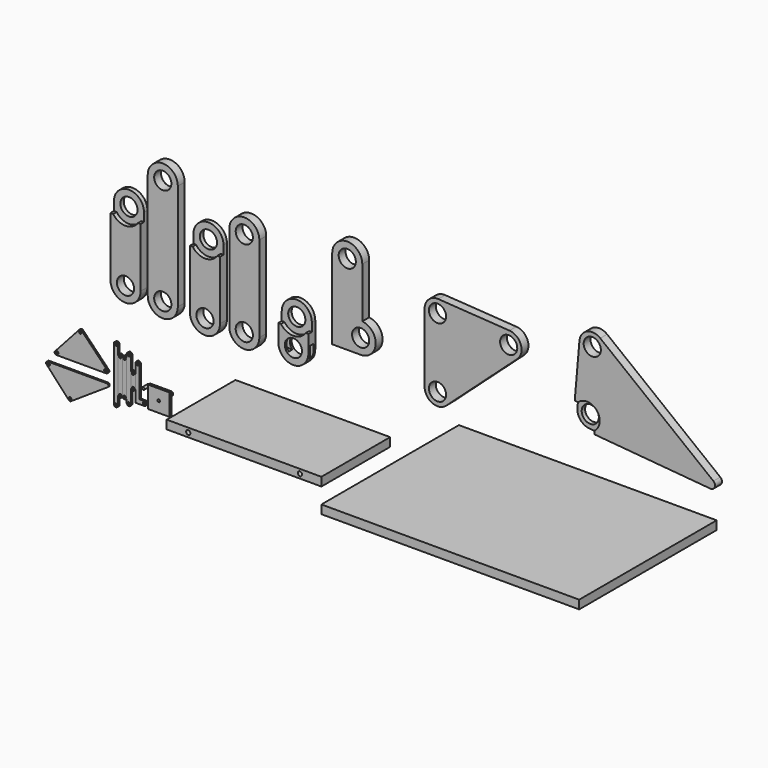
from build123d import *

# Parameters (mm, degrees)
F0_R           = 1.5
F1_DEPTH       = 2
F2_R           = 1.5
F3_DEPTH       = 2
F4_R           = 1.5
F5_DEPTH       = 2
F6_R           = 1.5
F7_DEPTH       = 2
F8_R           = 1.5
F9_DEPTH       = 2
F10_R          = 1.5
F11_DEPTH      = 2
F12_R          = 2
F13_R          = 1.5
F14_DEPTH      = 2
F15_R          = 2
F16_R          = 1.5
F17_DEPTH      = 2
F18_R          = 1.5
F19_DEPTH      = 6
F20_R          = 2.5
F21_DEPTH      = 15
F22_W          = 25
F22_H          = 25
F22_R          = 2.5
F23_DEPTH      = 3
F24_R          = 1.5
F25_DEPTH      = 4
F26_R          = 1.5
F27_DEPTH      = 8
F28_W          = 180
F28_H          = 100
F29_DEPTH      = 5
F29_DEPTH_BACK = 5
F30_R          = 2.5
F31_DEPTH      = 15
F32_W          = 300
F32_H          = 200
F33_DEPTH      = 10
F34_R          = 10
F35_DEPTH      = 10
F36_R          = 10
F37_DEPTH      = 10
F38_R          = 10
F39_DEPTH      = 10
F40_R          = 10
F41_DEPTH      = 10
F42_R          = 10
F43_DEPTH      = 10
F44_R          = 10
F45_DEPTH      = 10
F46_R          = 10
F47_DEPTH      = 10
F48_R          = 10
F49_DEPTH      = 10
F51_DEPTH      = 5
F53_DEPTH      = 5
F55_DEPTH      = 5
F57_DEPTH      = 5
F59_W          = 55.4324309552
F59_H          = 14
F60_DEPTH      = 2.5
F60_DEPTH_BACK = 2.5


# Not quite as in the source:
# - a pattern or mirror of a feature is missing from the dataset's text; its kind, count and spacing are read off the source's solid


with BuildPart() as f1:
    # F0 (on Front) → F1 (new body)
    with BuildSketch(Plane.XZ):
        with BuildLine():
            ThreePointArc((5, 7.5), (2.5, 10), (0, 7.5))
            Line((0, 7.5), (0, -7.5))
            ThreePointArc((0, -7.5), (2.5, -10), (5, -7.5))
            Line((5, -7.5), (5, 7.5))
        make_face()
        with Locations((2.5, -7.5)):
            Circle(F0_R, mode=Mode.SUBTRACT)
        with Locations((2.5, 7.5)):
            Circle(F0_R, mode=Mode.SUBTRACT)
    extrude(amount=F1_DEPTH)


with BuildPart() as f3:
    # F2 (on Front) → F3 (new body)
    with BuildSketch(Plane.XZ):
        with BuildLine():
            Line((0, -25), (0, 25))
            ThreePointArc((0, 25), (-2.5, 27.5), (-5, 25))
            Line((-5, 25), (-5, -25))
            ThreePointArc((-5, -25), (-2.5, -27.5), (0, -25))
        make_face()
        with Locations((-2.5, -25)):
            Circle(F2_R, mode=Mode.SUBTRACT)
        with Locations((-2.5, 25)):
            Circle(F2_R, mode=Mode.SUBTRACT)
    extrude(amount=F3_DEPTH)


with BuildPart() as f5:
    # F4 (on Front) → F5 (new body)
    with BuildSketch(Plane.XZ):
        with BuildLine():
            Line((-5, -19.65), (-5, 19.65))
            ThreePointArc((-5, 19.65), (-7.5, 22.15), (-10, 19.65))
            Line((-10, 19.65), (-10, -19.65))
            ThreePointArc((-10, -19.65), (-7.5, -22.15), (-5, -19.65))
        make_face()
        with Locations((-7.5, -19.65)):
            Circle(F4_R, mode=Mode.SUBTRACT)
        with Locations((-7.5, 19.65)):
            Circle(F4_R, mode=Mode.SUBTRACT)
    extrude(amount=F5_DEPTH)


with BuildPart() as f7:
    # F6 (on Front) → F7 (new body)
    with BuildSketch(Plane.XZ):
        with BuildLine():
            Line((-10, -19.7), (-10, 19.7))
            ThreePointArc((-10, 19.7), (-12.5, 22.2), (-15, 19.7))
            Line((-15, 19.7), (-15, -19.7))
            ThreePointArc((-15, -19.7), (-12.5, -22.2), (-10, -19.7))
        make_face()
        with Locations((-12.5, -19.7)):
            Circle(F6_R, mode=Mode.SUBTRACT)
        with Locations((-12.5, 19.7)):
            Circle(F6_R, mode=Mode.SUBTRACT)
    extrude(amount=F7_DEPTH)


with BuildPart() as f9:
    # F8 (on Front) → F9 (new body)
    with BuildSketch(Plane.XZ):
        with BuildLine():
            ThreePointArc((-15, 30.95), (-17.5, 33.45), (-20, 30.95))
            Line((-20, 30.95), (-20, -30.95))
            ThreePointArc((-20, -30.95), (-17.5, -33.45), (-15, -30.95))
            Line((-15, -30.95), (-15, 30.95))
        make_face()
        with Locations((-17.5, -30.95)):
            Circle(F8_R, mode=Mode.SUBTRACT)
        with Locations((-17.5, 30.95)):
            Circle(F8_R, mode=Mode.SUBTRACT)
    extrude(amount=F9_DEPTH)


with BuildPart() as f11:
    # F10 (on Front) → F11 (new body)
    with BuildSketch(Plane.XZ):
        Polygon((-58.9906042212, 33.4161580731), (-91.4263268434, -2.5), (-24.0840828044, -2.5), align=None)
        with Locations((-85.8, 0)):
            Circle(F10_R, mode=Mode.SUBTRACT)
        with Locations((-30, 0)):
            Circle(F10_R, mode=Mode.SUBTRACT)
        with Locations((-58.923655914, 29.7602440946)):
            Circle(F10_R, mode=Mode.SUBTRACT)
    extrude(amount=F11_DEPTH)

    # F12
    f12_edges = [f11.edges().sort_by_distance(p)[0] for p in [
        (-91.426327, -1, -2.5),
        (-24.084083, -1, -2.5),
        (-58.990604, -1, 33.416158),
    ]]
    fillet(f12_edges, radius=F12_R)


with BuildPart() as f14:
    # F13 (on Front) → F14 (new body)
    with BuildSketch(Plane.XZ):
        Polygon((-21.6868690575, -12.5), (-101.3912973376, -12.5), (-71.2712075502, -45.2882004463), align=None)
        with Locations((-70.8721461187, -42.0271654387)):
            Circle(F13_R, mode=Mode.SUBTRACT)
        with Locations((-95.7, -15)):
            Circle(F13_R, mode=Mode.SUBTRACT)
    extrude(amount=F14_DEPTH)

    # F15
    f15_edges = [f14.edges().sort_by_distance(p)[0] for p in [
        (-101.391297, -1, -12.5),
        (-71.271208, -1, -45.2882),
        (-21.686869, -1, -12.5),
    ]]
    fillet(f15_edges, radius=F15_R)


with BuildPart() as f17:
    # F16 (on Front) → F17 (new body)
    with BuildSketch(Plane.XZ):
        with BuildLine():
            Line((10, -16.5), (10, 19))
            ThreePointArc((10, 19), (7.5, 21.5), (5, 19))
            Line((5, 19), (5, -21.5))
            Line((5, -21.5), (15.3, -21.5))
            ThreePointArc((15.3, -21.5), (17.8, -19), (15.3, -16.5))
            Line((15.3, -16.5), (10, -16.5))
        make_face()
        with Locations((15.3, -19)):
            Circle(F16_R, mode=Mode.SUBTRACT)
        with Locations((7.5, 19)):
            Circle(F16_R, mode=Mode.SUBTRACT)
    extrude(amount=F17_DEPTH)


with BuildPart() as f19:
    # F18 (on Front) → F19 (new body)
    with BuildSketch(Plane.XZ):
        with Locations((24.9495524913, 0)):
            Circle(F18_R)
    extrude(amount=F19_DEPTH)


with BuildPart() as f21:
    # F20 (on Front) → F21 (new body)
    with BuildSketch(Plane.XZ):
        with Locations((45, 0)):
            Circle(F20_R)
    extrude(amount=F21_DEPTH)

    # F22 (on face) → F23 (join)
    with BuildSketch(Plane.XZ.offset(15)):
        with Locations((45, 0)):
            Rectangle(F22_W, F22_H)
        with Locations((45, 0)):
            Circle(F22_R, mode=Mode.SUBTRACT)
        with Locations((45, 0)):
            Circle(F22_R)
    extrude(amount=F23_DEPTH)

    # F24 (on face) → F25 (cut)
    with BuildSketch(Plane.XZ.offset(18)):
        with Locations((45, 0)):
            Circle(F24_R)
    extrude(amount=-F25_DEPTH, mode=Mode.SUBTRACT)


with BuildPart() as f27:
    # F26 (on Front) → F27 (new body)
    with BuildSketch(Plane.XZ):
        with Locations((18.9495524913, 0)):
            Circle(F26_R)
    extrude(amount=F27_DEPTH)


with BuildPart() as f29:
    # F28 (on Top) → F29 (new body, two sides)
    with BuildSketch(Plane.XY) as f29_sk:
        with Locations((170, 0)):
            Rectangle(F28_W, F28_H)
    extrude(amount=F29_DEPTH)
    extrude(f29_sk.sketch, amount=-F29_DEPTH_BACK)

    # F30 (on face) → F31 (cut)
    with BuildSketch(Plane.XZ.offset(50)):
        with Locations((105, 0)):
            Circle(F30_R)
        with Locations((235, 0)):
            Circle(F30_R)
    f31 = extrude(amount=-F31_DEPTH, mode=Mode.SUBTRACT)

    # F31_copies: F31 across plane
    add(f31.mirror(Plane.ZX), mode=Mode.SUBTRACT)


with BuildPart() as f33:
    # F32 (on Top) → F33 (new body)
    with BuildSketch(Plane.XY):
        with Locations((450, 0)):
            Rectangle(F32_W, F32_H)
    extrude(amount=F33_DEPTH)


with BuildPart() as f35:
    # F34 (on Front) → F35 (new body)
    with BuildSketch(Plane.XZ):
        with BuildLine():
            Line((17.5, 100), (17.5, 178.8))
            ThreePointArc((17.5, 178.8), (0, 196.3), (-17.5, 178.8))
            Line((-17.5, 178.8), (-17.5, 100))
            ThreePointArc((-17.5, 100), (0, 82.5), (17.5, 100))
        make_face()
        with Locations((0, 100)):
            Circle(F34_R, mode=Mode.SUBTRACT)
        with Locations((0, 178.8)):
            Circle(F34_R, mode=Mode.SUBTRACT)
    extrude(amount=F35_DEPTH)

    # F50 (on face) → F51 (cut)
    with BuildSketch(Plane.XZ.offset(10)):
        with BuildLine():
            Line((-17.5, 168.8), (-14.3614066163, 168.8))
            ThreePointArc((-14.3614066163, 168.8), (0, 161.3), (14.3614066163, 168.8))
            Line((14.3614066163, 168.8), (17.5, 168.8))
            Line((17.5, 168.8), (17.5, 178.8))
            ThreePointArc((17.5, 178.8), (0, 196.3), (-17.5, 178.8))
            Line((-17.5, 178.8), (-17.5, 168.8))
        make_face()
    extrude(amount=-F51_DEPTH, mode=Mode.SUBTRACT)


with BuildPart() as f37:
    # F36 (on Front) → F37 (new body)
    with BuildSketch(Plane.XZ):
        with BuildLine():
            Line((25.8714240789, 221.8801135302), (25.8714240789, 98.0801135302))
            ThreePointArc((25.8714240789, 98.0801135302), (43.3714240789, 80.5801135302), (60.8714240789, 98.0801135302))
            Line((60.8714240789, 98.0801135302), (60.8714240789, 221.8801135302))
            ThreePointArc((60.8714240789, 221.8801135302), (43.3714240789, 239.3801135302), (25.8714240789, 221.8801135302))
        make_face()
        with Locations((43.3714240789, 98.0801135302)):
            Circle(F36_R, mode=Mode.SUBTRACT)
        with Locations((43.3714240789, 221.8801135302)):
            Circle(F36_R, mode=Mode.SUBTRACT)
    extrude(amount=F37_DEPTH)


with BuildPart() as f39:
    # F38 (on Front) → F39 (new body)
    with BuildSketch(Plane.XZ):
        with BuildLine():
            Line((110.0058871508, 96.7913018195), (110.0058871508, 175.3913018195))
            ThreePointArc((110.0058871508, 175.3913018195), (92.5058871508, 192.8913018195), (75.0058871508, 175.3913018195))
            Line((75.0058871508, 175.3913018195), (75.0058871508, 96.7913018195))
            ThreePointArc((75.0058871508, 96.7913018195), (92.5058871508, 79.2913018195), (110.0058871508, 96.7913018195))
        make_face()
        with Locations((92.5058871508, 96.7913018195)):
            Circle(F38_R, mode=Mode.SUBTRACT)
        with Locations((92.5058871508, 175.3913018195)):
            Circle(F38_R, mode=Mode.SUBTRACT)
    extrude(amount=F39_DEPTH)

    # F54 (on face) → F55 (cut)
    with BuildSketch(Plane.XZ.offset(10)):
        with BuildLine():
            Line((75.0058871508, 165.3913018195), (78.1444805344, 165.3913018195))
            ThreePointArc((78.1444805344, 165.3913018195), (92.5058871508, 157.8913018195), (106.8672937671, 165.3913018195))
            Line((106.8672937671, 165.3913018195), (110.0058871508, 165.3913018195))
            Line((110.0058871508, 165.3913018195), (110.0058871508, 175.3913018195))
            ThreePointArc((110.0058871508, 175.3913018195), (92.5058871508, 192.8913018195), (75.0058871508, 175.3913018195))
            Line((75.0058871508, 175.3913018195), (75.0058871508, 165.3913018195))
        make_face()
    extrude(amount=-F55_DEPTH, mode=Mode.SUBTRACT)


with BuildPart() as f41:
    # F40 (on Front) → F41 (new body)
    with BuildSketch(Plane.XZ):
        with BuildLine():
            Line((155.7446885109, 97.4593386054), (155.7446885109, 197.4593386054))
            ThreePointArc((155.7446885109, 197.4593386054), (138.2446885109, 214.9593386054), (120.7446885109, 197.4593386054))
            Line((120.7446885109, 197.4593386054), (120.7446885109, 97.4593386054))
            ThreePointArc((120.7446885109, 97.4593386054), (138.2446885109, 79.9593386054), (155.7446885109, 97.4593386054))
        make_face()
        with Locations((138.2446885109, 97.4593386054)):
            Circle(F40_R, mode=Mode.SUBTRACT)
        with Locations((138.2446885109, 197.4593386054)):
            Circle(F40_R, mode=Mode.SUBTRACT)
    extrude(amount=F41_DEPTH)


with BuildPart() as f43:
    # F42 (on Front) → F43 (new body)
    with BuildSketch(Plane.XZ):
        with BuildLine():
            Line((212.8325867653, 99.6766347766), (212.8325867653, 129.6766347766))
            ThreePointArc((212.8325867653, 129.6766347766), (195.3325867653, 147.1766347766), (177.8325867653, 129.6766347766))
            Line((177.8325867653, 129.6766347766), (177.8325867653, 99.6766347766))
            ThreePointArc((177.8325867653, 99.6766347766), (195.3325867653, 82.1766347766), (212.8325867653, 99.6766347766))
        make_face()
        with Locations((195.3325867653, 99.6766347766)):
            Circle(F42_R, mode=Mode.SUBTRACT)
        with Locations((195.3325867653, 129.6766347766)):
            Circle(F42_R, mode=Mode.SUBTRACT)
    extrude(amount=F43_DEPTH)

    # F52 (on face) → F53 (cut)
    with BuildSketch(Plane.XZ.offset(10)):
        with BuildLine():
            Line((177.8325867653, 119.6766347766), (180.9711801489, 119.6766347766))
            ThreePointArc((180.9711801489, 119.6766347766), (195.3325867653, 112.1766347766), (209.6939933816, 119.6766347766))
            Line((209.6939933816, 119.6766347766), (212.8325867653, 119.6766347766))
            Line((212.8325867653, 119.6766347766), (212.8325867653, 129.6766347766))
            ThreePointArc((212.8325867653, 129.6766347766), (195.3325867653, 147.1766347766), (177.8325867653, 129.6766347766))
            Line((177.8325867653, 129.6766347766), (177.8325867653, 119.6766347766))
        make_face()
    extrude(amount=-F53_DEPTH, mode=Mode.SUBTRACT)

    # F59 (on offset) → F60 (cut, two sides)
    with BuildSketch(Plane.XZ.offset(5)) as f60_sk:
        with Locations((198.0529725552, 99.6766347766)):
            Rectangle(F59_W, F59_H)
    extrude(amount=-F60_DEPTH, mode=Mode.SUBTRACT)
    extrude(f60_sk.sketch, amount=F60_DEPTH_BACK, mode=Mode.SUBTRACT)


with BuildPart() as f45:
    # F44 (on Front) → F45 (new body)
    with BuildSketch(Plane.XZ):
        with BuildLine():
            Line((275.5794075251, 153.0540936323), (275.5794075251, 211.6575422499))
            ThreePointArc((275.5794075251, 211.6575422499), (258.0794075251, 229.1575422499), (240.5794075251, 211.6575422499))
            Line((240.5794075251, 211.6575422499), (240.5794075251, 118.1575422499))
            Line((240.5794075251, 118.1575422499), (273.6794075251, 118.1575422499))
            ThreePointArc((273.6794075251, 118.1575422499), (291.1535262323, 134.7061351845), (275.5794075251, 153.0540936323))
        make_face()
        with Locations((273.6794075251, 135.6575422499)):
            Circle(F44_R, mode=Mode.SUBTRACT)
        with Locations((258.0794075251, 211.6575422499)):
            Circle(F44_R, mode=Mode.SUBTRACT)
    extrude(amount=F45_DEPTH)


with BuildPart() as f47:
    # F46 (on Front) → F47 (new body)
    with BuildSketch(Plane.XZ):
        with BuildLine():
            Line((446.9155081679, 199.2951546795), (364.0914871964, 204.697149692))
            ThreePointArc((364.0914871964, 204.697149692), (352.8595895218, 200.6752758555), (348.1152230375, 189.7289531309))
            Line((348.1152230375, 189.7289531309), (348.1152230375, 109.5289531309))
            ThreePointArc((348.1152230375, 109.5289531309), (357.0243458187, 95.8212467325), (373.1687183315, 98.3966922476))
            Line((373.1687183315, 98.3966922476), (455.992739303, 173.1946972351))
            ThreePointArc((455.992739303, 173.1946972351), (460.1068961821, 189.2541918151), (446.9155081679, 199.2951546795))
        make_face()
        with Locations((363.1152230375, 109.5289531309)):
            Circle(F46_R, mode=Mode.SUBTRACT)
        with Locations((363.1152230375, 189.7289531309)):
            Circle(F46_R, mode=Mode.SUBTRACT)
        with Locations((445.939244009, 184.3269581184)):
            Circle(F46_R, mode=Mode.SUBTRACT)
    extrude(amount=F47_DEPTH)


with BuildPart() as f49:
    # F48 (on Front) → F49 (new body)
    with BuildSketch(Plane.XZ):
        with BuildLine():
            Line((684.2155163305, 122.3244659342), (552.4956518054, 225.8431882922))
            ThreePointArc((552.4956518054, 225.8431882922), (537.2594333344, 227.8113305554), (528.2829203377, 215.3438467802))
            Line((528.2829203377, 215.3438467802), (521.9491563461, 142.2176310043))
            ThreePointArc((521.9491563461, 142.2176310043), (525.4109121872, 131.2714812263), (535.5988399532, 125.9792155205))
            Line((535.5988399532, 125.9792155205), (680.6945003769, 113.4118802689))
            ThreePointArc((680.6945003769, 113.4118802689), (685.776216628, 116.5560928863), (684.2155163305, 122.3244659342))
        make_face()
        with Locations((536.8932058915, 140.923265066)):
            Circle(F48_R, mode=Mode.SUBTRACT)
        with Locations((543.2269698832, 214.0494808419)):
            Circle(F48_R, mode=Mode.SUBTRACT)
    extrude(amount=F49_DEPTH)

    # F56 (on face) → F57 (cut)
    with BuildSketch(Plane.XZ.offset(10)):
        with BuildLine():
            Line((522.8120669716, 152.1803307013), (521.9491563461, 142.2176310043))
            ThreePointArc((521.9491563461, 142.2176310043), (525.4109121872, 131.2714812263), (535.5988399532, 125.9792155205))
            Line((535.5988399532, 125.9792155205), (545.5615396502, 125.116304895))
            Line((545.5615396502, 125.116304895), (545.8911421799, 128.9217175595))
            ThreePointArc((545.8911421799, 128.9217175595), (548.3754995959, 150.5750489057), (526.6174796362, 151.8507281716))
            Line((526.6174796362, 151.8507281716), (522.8120669716, 152.1803307013))
        make_face()
    extrude(amount=-F57_DEPTH, mode=Mode.SUBTRACT)


solid = Compound([f1.part, f3.part, f5.part, f7.part, f9.part, f11.part, f14.part, f17.part, f19.part, f21.part, f27.part, f29.part, f33.part, f35.part, f37.part, f39.part, f41.part, f43.part, f45.part, f47.part, f49.part])
